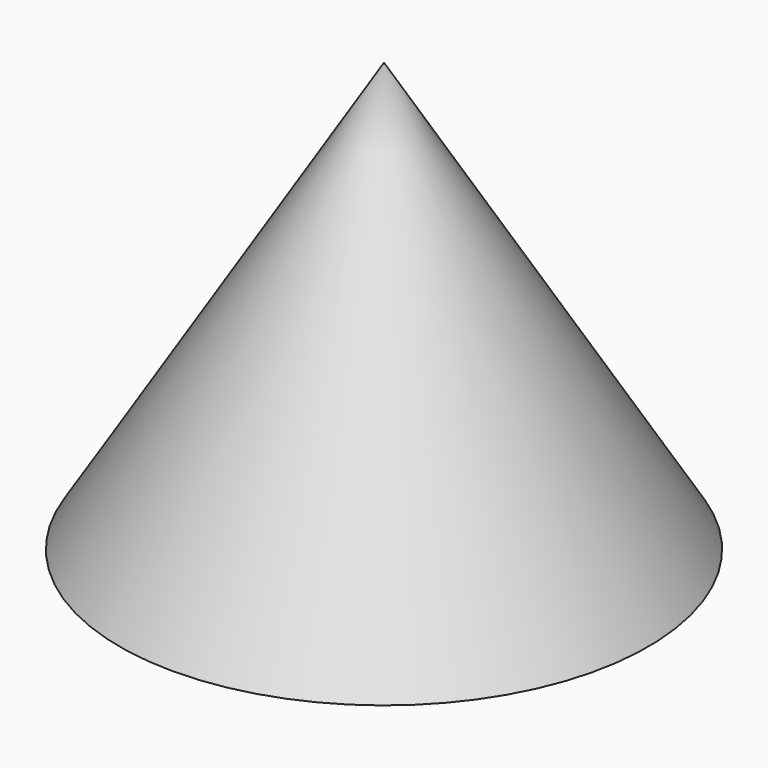
from build123d import *


# Not quite as in the source:
# - the program builds the solid bodies; features that only make, move or delete a surface that nothing else refers to are left out


with BuildPart() as f1:
    # F0 (on Right) → F1 (revolve)
    with BuildSketch(Plane.YZ):
        Polygon((-10.4160485789, -24.9800812453), (-38.2536277175, 20.1868545264), (-38.2536277175, -24.9800812453), align=None)
    revolve(axis=Axis((0, -38.2536277175, -2.3966133595), (0, 0, -1)))


solid = f1.part
